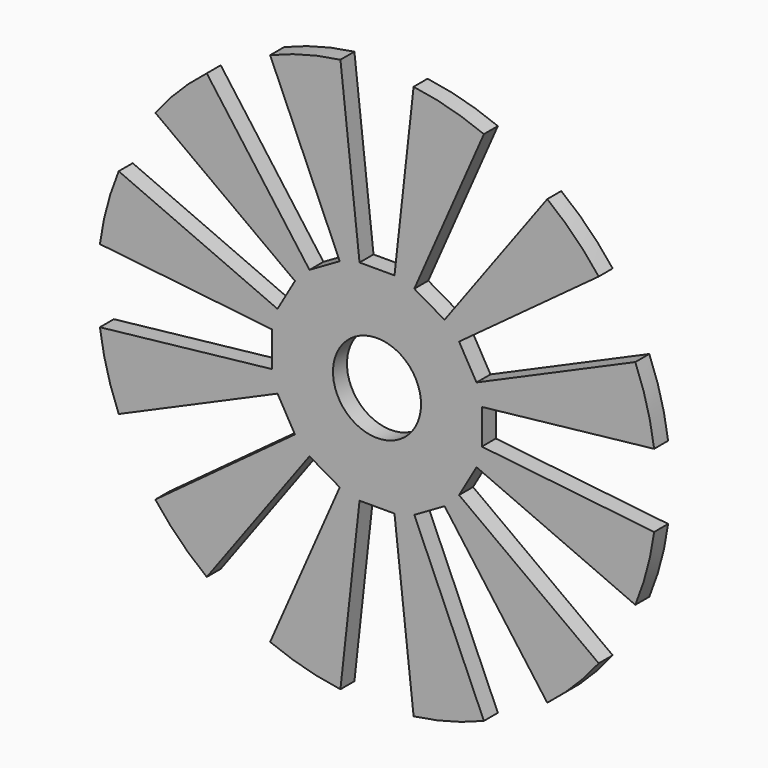
from build123d import *

# Parameters (mm, degrees)
F0_R            = 25.4
F0_R_2          = 4
F1_DEPTH        = 0.79375
F3_DEPTH        = 25.4
F3_COPIES_COUNT = 12


# Not quite as in the source:
# - a pattern or mirror of a feature is missing from the dataset's text; its kind, count and spacing are read off the source's solid


with BuildPart() as f1:
    # F0 (on Front) → F1 (new body, symmetric)
    with BuildSketch(Plane.XZ):
        Circle(F0_R)
        Circle(F0_R_2, mode=Mode.SUBTRACT)
    extrude(amount=F1_DEPTH, both=True)

    # F2 (on face) → F3 (cut)
    with BuildSketch(Plane.XZ.offset(0.79375)):
        Polygon((-1.5875, 9.525), (1.5875, 9.525), (3.3247541667, 25.1814616282), (0, 29.9078127353), (-3.3247541667, 25.1814616282), align=None)
    f3 = extrude(amount=-F3_DEPTH, mode=Mode.SUBTRACT)

    # F3_copies: F3 ×12 about axis
    f3_copies_axis = Axis((0, 0, 0), (0, 1, 0))
    for i in range(1, F3_COPIES_COUNT):
        add(f3.rotate(f3_copies_axis, i * 360 / F3_COPIES_COUNT), mode=Mode.SUBTRACT)


solid = f1.part
